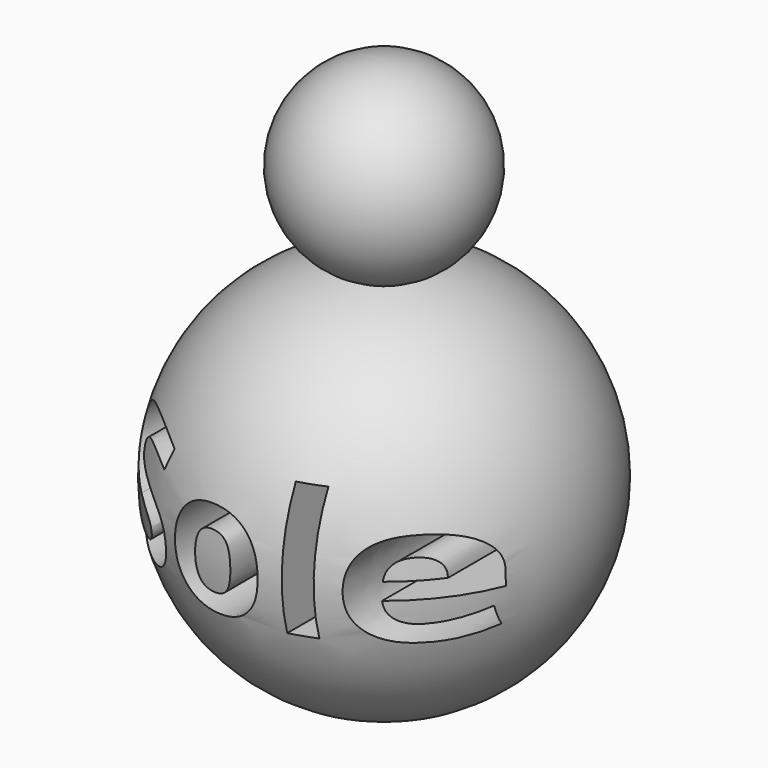
from build123d import *

# Parameters (mm, degrees)
F2_TEXT_SIZE = 36.9961839169
F3_DEPTH     = 55.118


# Not quite as in the source:
# - Text() gives the source's letters only with a copy of the font that has no kerning and outlines rounded to 1/6400 em; it was checked with that copy


with BuildPart() as f1:
    # F0 (on Front) → F1 (revolve)
    with BuildSketch(Plane.XZ):
        with BuildLine():
            ThreePointArc((0, 79.8036095078), (-19.9326811729, 63.8599667378), (-8.7568874593, 40.9119132607))
            ThreePointArc((-8.7568874593, 40.9119132607), (-4.4880594738, 39.4392260911), (0, 38.9402050202))
            Line((0, 38.9402050202), (0, 79.8036095078))
        make_face()
        with BuildLine():
            ThreePointArc((0, 38.9402050202), (-4.4880594738, 39.4392260911), (-8.7568874593, 40.9119132607))
            ThreePointArc((-8.7568874593, 40.9119132607), (-41.606276835, -4.4028913859), (0, -41.8385913317))
            Line((0, -41.8385913317), (0, 38.9402050202))
        make_face()
    revolve(axis=Axis((0, 0, 18.982509088), (0, 0, -1)))

    # F2 (on Front) → F3 (cut)
    with BuildSketch(Plane.XZ):
        with Locations((-35.9755977988, -10.9044704586)):
            Text('Sole', F2_TEXT_SIZE, font='Open Sans', font_style=FontStyle.BOLD, text_align=(TextAlign.LEFT, TextAlign.BOTTOM))
    extrude(amount=F3_DEPTH, mode=Mode.SUBTRACT)


solid = f1.part
